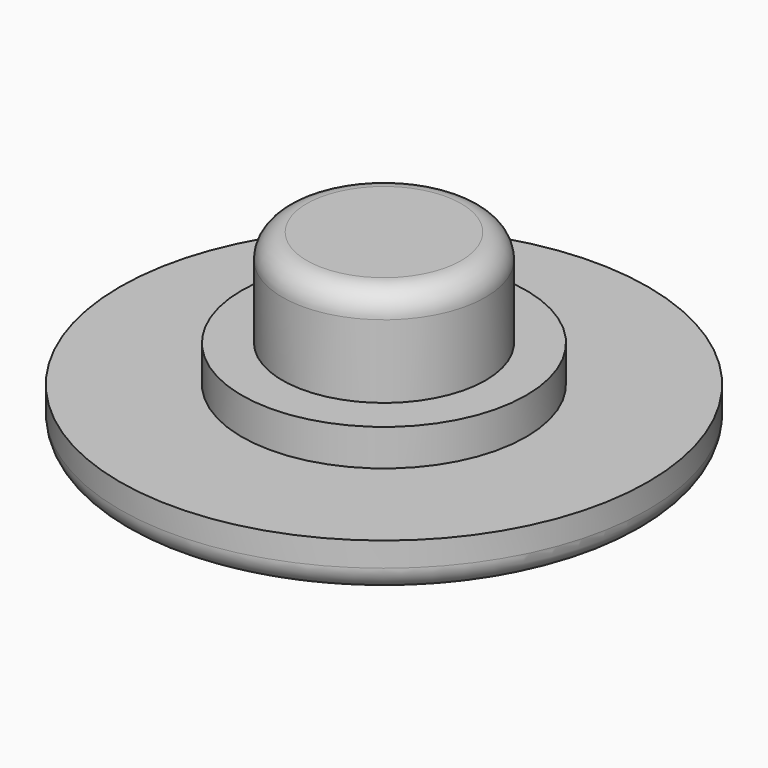
from build123d import *

# Parameters (mm, degrees)
F0_R     = 6.5
F0_R_2   = 3.5
F4_DEPTH = 1.2
F0_R_3   = 2.5
F5_DEPTH = 2.1
F6_DEPTH = 4.5
F7_R     = 0.6


# Not quite as in the source:
# - a feature names something its author has since deleted; it is built from what else it names


with BuildPart() as f4:
    # F0 (on Top) → F4 (new body)
    with BuildSketch(Plane.XY):
        Circle(F0_R)
        Circle(F0_R_2, mode=Mode.SUBTRACT)
    extrude(amount=F4_DEPTH)

    # F0 (on Top) → F5 (join)
    with BuildSketch(Plane.XY):
        Circle(F0_R_2)
        Circle(F0_R_3, mode=Mode.SUBTRACT)
    extrude(amount=F5_DEPTH)

    # F0 (on Top) → F6 (join)
    with BuildSketch(Plane.XY):
        Circle(F0_R_3)
    extrude(amount=F6_DEPTH)

    # F7
    f7_edges = [f4.edges().sort_by_distance(p)[0] for p in [
        (-2.5, 0, 4.5),
        (-6.5, 0, 0),
    ]]
    fillet(f7_edges, radius=F7_R)


solid = f4.part
